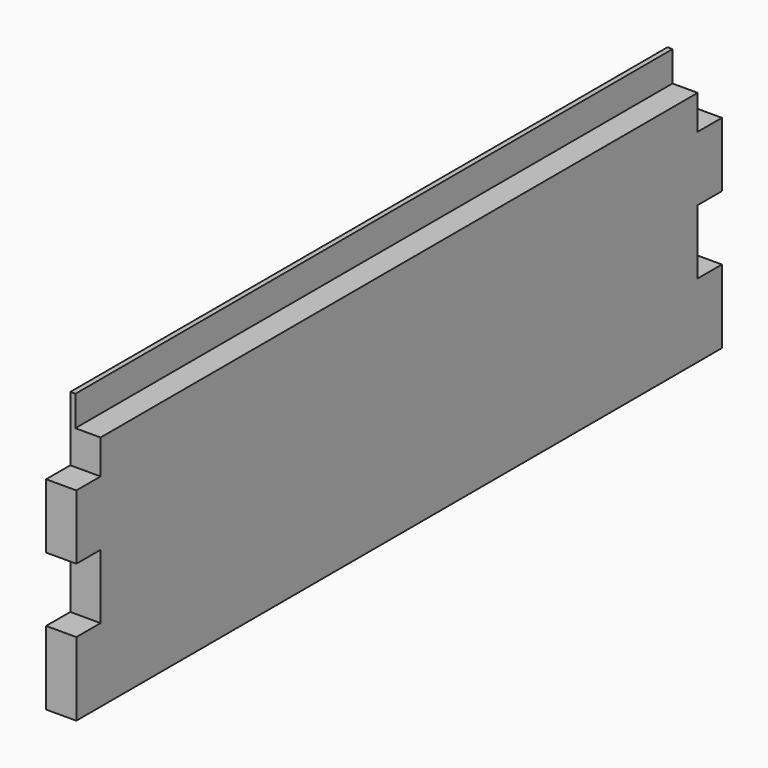
from build123d import *

# Parameters (mm, degrees)
F1_DEPTH = 19.05
F2_W     = 469.9
F2_H     = 19.05
F3_DEPTH = 15.875


# Not quite as in the source:
# - a feature names something its author has since deleted; it is built from what else it names


with BuildPart() as f1:
    # F0 (on Right) → F1 (new body)
    with BuildSketch(Plane.YZ):
        Polygon((-599.0287601471, -207.9838508803), (-618.0787601471, -207.9838508803), (-618.0787601471, -248.6238508803), (-599.0287601471, -248.6238508803), (-599.0287601471, -289.2638508803), (-618.0787601471, -289.2638508803), (-618.0787601471, -335.6188508803), (-110.0787601471, -335.6188508803), (-110.0787601471, -289.2638508803), (-129.1287601471, -289.2638508803), (-129.1287601471, -248.6238508803), (-110.0787601471, -248.6238508803), (-110.0787601471, -207.9838508803), (-129.1287601471, -207.9838508803), (-129.1287601471, -167.3438508803), (-599.0287601471, -167.3438508803), align=None)
    extrude(amount=F1_DEPTH)

    # F2 (on face) → F3 (cut)
    with BuildSketch(Plane.YZ.offset(19.05)):
        with Locations((-364.0787601471, -176.8688508803)):
            Rectangle(F2_W, F2_H)
    extrude(amount=-F3_DEPTH, mode=Mode.SUBTRACT)


solid = f1.part
